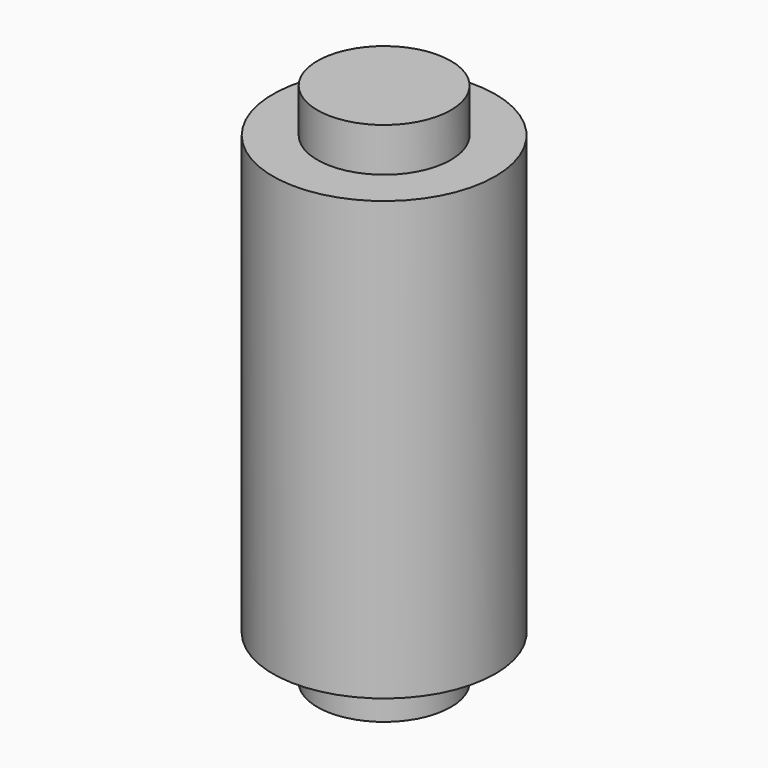
from build123d import *

# Parameters (mm, degrees)
F0_R     = 152.4
F1_DEPTH = 100
F2_R     = 254
F2_R_2   = 152.4
F3_DEPTH = 1000
F4_R     = 152.4
F5_DEPTH = 100


with BuildPart() as f1:
    # F0 (on Top) → F1 (new body)
    with BuildSketch(Plane.XY):
        Circle(F0_R)
    extrude(amount=F1_DEPTH)

    # F2 (on face) → F3 (join)
    with BuildSketch(Plane(origin=(0, 0, 0), x_dir=(1, 0, 0), z_dir=(0, 0, -1))):
        Circle(F2_R)
        Circle(F2_R_2, mode=Mode.SUBTRACT)
        Circle(F2_R_2)
    extrude(amount=F3_DEPTH)

    # F4 (on face) → F5 (join)
    with BuildSketch(Plane(origin=(0, 0, -1000), x_dir=(1, 0, 0), z_dir=(0, 0, -1))):
        Circle(F4_R)
    extrude(amount=F5_DEPTH)


solid = f1.part
